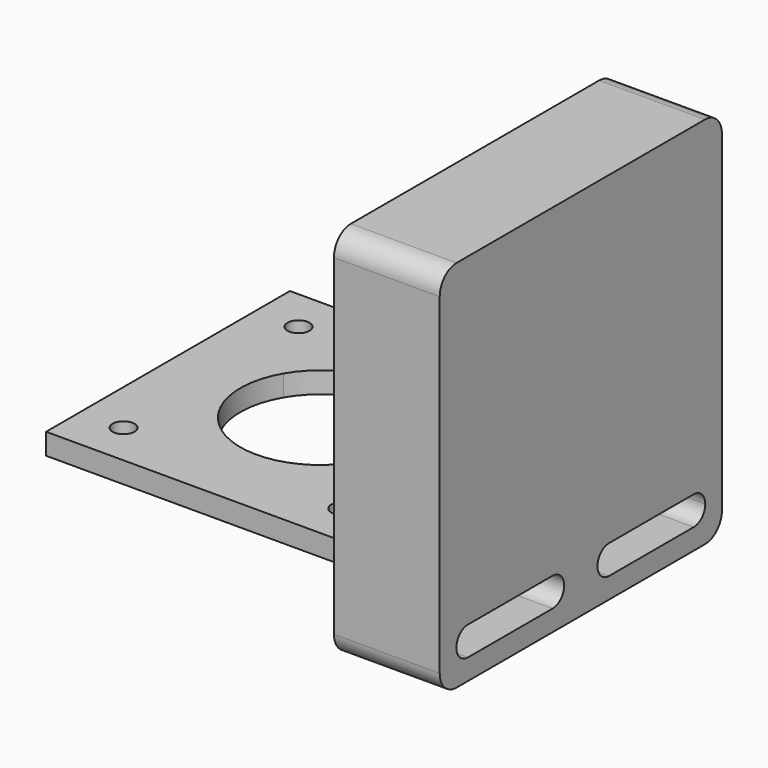
from build123d import *

# Parameters (mm, degrees)
F0_W     = 43.2
F0_H     = 43.2
F0_R     = 1.55
F1_DEPTH = 3
F2_W     = 50
F2_H     = 53
F2_R     = 2.3311267536
F3_DEPTH = 15
F4_R     = 3


with BuildPart() as f1:
    # F0 (on Top) → F1 (new body)
    with BuildSketch(Plane.XY):
        Rectangle(F0_W, F0_H)
        with Locations((-15.5, -15.5)):
            Circle(F0_R, mode=Mode.SUBTRACT)
        with Locations((15.5, -15.5)):
            Circle(F0_R, mode=Mode.SUBTRACT)
        with Locations((-15.5, 15.5)):
            Circle(F0_R, mode=Mode.SUBTRACT)
        with BuildLine():
            ThreePointArc((10.6885137593, 3.8181374539), (11.1834058133, 1.9375072686), (11.35, 0))
            ThreePointArc((11.35, 0), (9.6645780725, -5.951338562), (5.1088668406, -10.135185228))
            ThreePointArc((5.1088668406, -10.135185228), (-8.2600200355, -7.7842513457), (-9.8146512505, 5.7004491779))
            ThreePointArc((-9.8146512505, 5.7004491779), (-2.1377646428, 11.1468588549), (7.0093744434, 8.9269910895))
            ThreePointArc((7.0093744434, 8.9269910895), (9.2102610211, 6.6327665362), (10.6885137593, 3.8181374539))
        make_face(mode=Mode.SUBTRACT)
        with Locations((15.5, 15.5)):
            Circle(F0_R, mode=Mode.SUBTRACT)
    extrude(amount=F1_DEPTH)


with BuildPart() as f3:
    # F2 (on face) → F3 (new body)
    with BuildSketch(Plane.YZ.offset(21.6)):
        with Locations((0.4, 16.5)):
            Rectangle(F2_W, F2_H)
        Circle(F2_R, mode=Mode.SUBTRACT)
        with BuildLine():
            ThreePointArc((-19.6, -7.05), (-21.65, -5), (-19.6, -2.95))
            Line((-19.6, -2.95), (-4.6, -2.95))
            Line((-4.6, -2.95), (5.4, -2.95))
            Line((5.4, -2.95), (20.4, -2.95))
            ThreePointArc((20.4, -2.95), (21.8495689014, -3.5504310986), (22.45, -5))
            ThreePointArc((22.45, -5), (21.8495689014, -6.4495689014), (20.4, -7.05))
            Line((20.4, -7.05), (5.4, -7.05))
            Line((5.4, -7.05), (-4.6, -7.05))
            Line((-4.6, -7.05), (-19.6, -7.05))
        make_face(mode=Mode.SUBTRACT)
        with BuildLine():
            Line((5.4, -2.95), (-4.6, -2.95))
            ThreePointArc((-4.6, -2.95), (-2.55, -5), (-4.6, -7.05))
            Line((-4.6, -7.05), (5.4, -7.05))
            ThreePointArc((5.4, -7.05), (3.35, -5), (5.4, -2.95))
        make_face()
        with BuildLine():
            ThreePointArc((-2.3311267536, 0), (0, -2.3311267536), (2.3311267536, 0))
            Line((2.3311267536, 0), (-2.3311267536, 0))
        make_face()
        with BuildLine():
            Line((-2.3311267536, 0), (2.3311267536, 0))
            ThreePointArc((2.3311267536, 0), (0, 2.3311267536), (-2.3311267536, 0))
        make_face()
    extrude(amount=F3_DEPTH)

    # F4
    f4_edges = [f3.edges().sort_by_distance(p)[0] for p in [
        (29.1, 25.4, -10),
        (29.1, -24.6, -10),
        (29.1, 25.4, 43),
        (29.1, -24.6, 43),
    ]]
    fillet(f4_edges, radius=F4_R)


solid = Compound([f1.part, f3.part])
